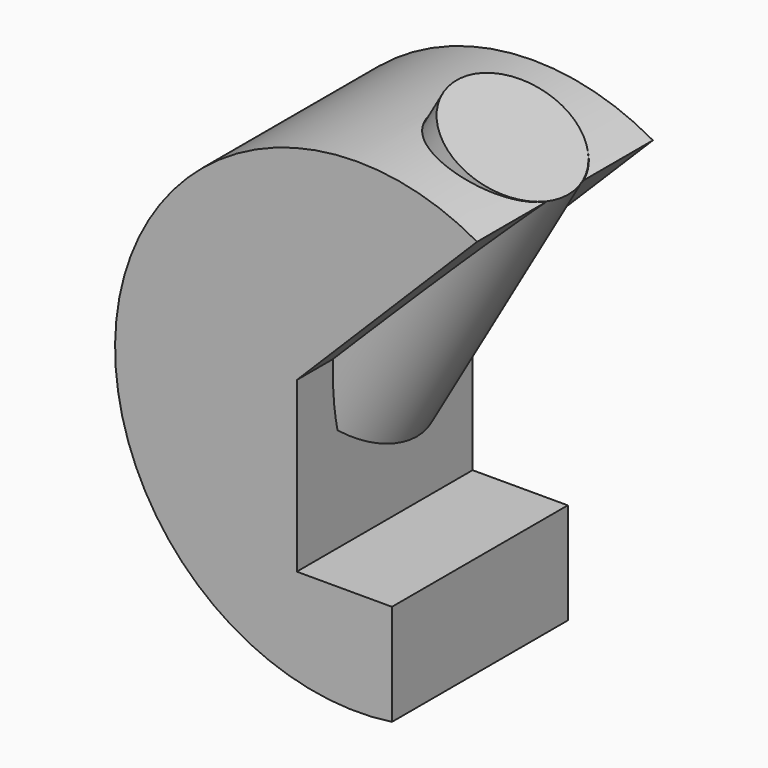
from build123d import *

# Parameters (mm, degrees)
F1_DEPTH  = 12.7
F3_R      = 7.5
F4_DEPTH  = 35
F6_DEPTH  = 25
F8_R      = 6.25
F9_DEPTH  = 8
F10_R     = 7.45
F11_DEPTH = 35


with BuildPart() as f1:
    # F0 (on Front) → F1 (new body, symmetric)
    with BuildSketch(Plane.XZ):
        with BuildLine():
            Line((-7, 3.5), (13.8402462006, 24.3402462006))
            ThreePointArc((13.8402462006, 24.3402462006), (-27.5127031952, 5.2010732444), (4, -27.7128129211))
            Line((4, -27.7128129211), (4, -16))
            Line((4, -16), (-7, -16))
            Line((-7, -16), (-7, 3.5))
        make_face()
    extrude(amount=F1_DEPTH, both=True)

    # F3 (on face) → F4 (cut)
    with BuildSketch(Plane(origin=(13.9996973222, 0, 24.2481870526), x_dir=(0.8660254038, 0, -0.5), z_dir=(-0.5, 0, -0.8660254038))):
        with Locations((-7.1841182959, 0)):
            Circle(F3_R)
    extrude(amount=F4_DEPTH, mode=Mode.SUBTRACT)

    # F5 (on face) → F6 (cut)
    with BuildSketch(Plane(origin=(-3.5003026778, 0, -6.0627020798), x_dir=(0.8660254038, 0, -0.5), z_dir=(0.5, 0, 0.8660254038))):
        with BuildLine():
            Line((-4.0411023821, -2.474156617), (-4.0411023821, 2.474156617))
            ThreePointArc((-4.0411023821, 2.474156617), (-11.1841182959, 0), (-4.0411023821, -2.474156617))
        make_face()
        with BuildLine():
            ThreePointArc((-4.0411023821, -2.474156617), (-3.4044315592, -1.3091860725), (-3.1841182959, 0))
            ThreePointArc((-3.1841182959, 0), (-3.4044315592, 1.3091860725), (-4.0411023821, 2.474156617))
            Line((-4.0411023821, 2.474156617), (-4.0411023821, -2.474156617))
        make_face()
    extrude(amount=-F6_DEPTH, mode=Mode.SUBTRACT)

    # F8 (on face) → F9 (cut)
    with BuildSketch(Plane(origin=(-14.2003026778, 0, -24.5956457208), x_dir=(0.8660254038, 0, -0.5), z_dir=(-0.5, 0, -0.8660254038))):
        with Locations((-7.1841182959, 0)):
            Circle(F8_R)
    extrude(amount=-F9_DEPTH, mode=Mode.SUBTRACT)


with BuildPart() as f11:
    # F10 (on face) → F11 (new body)
    with BuildSketch(Plane(origin=(-3.5003026778, 0, -6.0627020798), x_dir=(0.8660254038, 0, -0.5), z_dir=(0.5, 0, 0.8660254038))):
        with Locations((-7.1841182959, 0)):
            Circle(F10_R)
    extrude(amount=F11_DEPTH)


solid = Compound([f1.part, f11.part])
